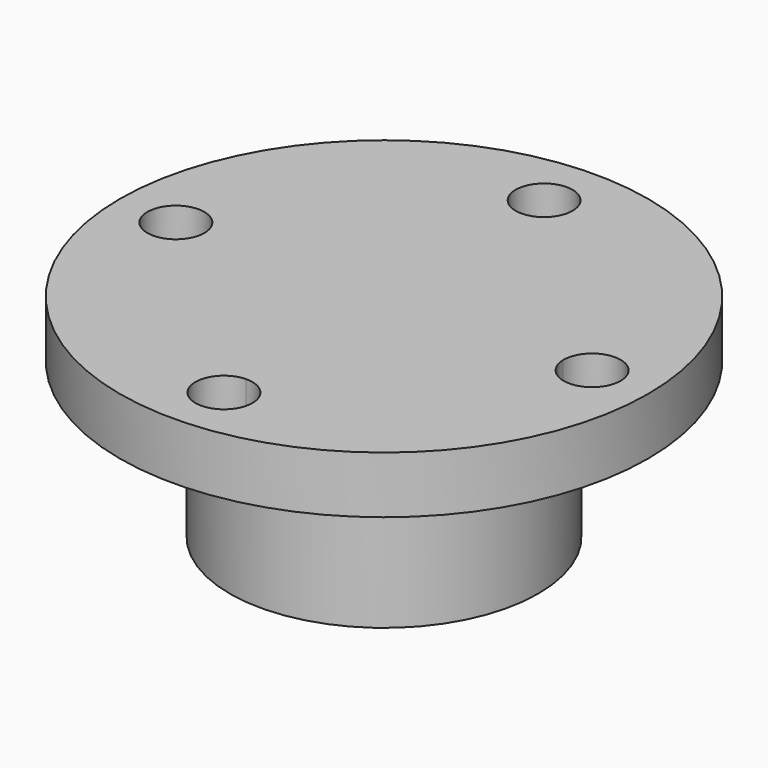
from build123d import *

# Parameters (mm, degrees)
F0_R         = 12.0396
F0_R_2       = 10.7696
F1_DEPTH     = 12.065
F2_R         = 20.6121
F3_DEPTH     = 4.445
F5_DEPTH     = 16.511
F6_S5_R      = 12.0396
F6_T6_DEPTH  = 7
F6_S11_R     = 12.0396
F6_T12_DEPTH = 7
F6_S17_R     = 12.0396
F6_T18_DEPTH = 7
F6_S23_R     = 12.0396
F6_T24_DEPTH = 7
F7_W         = 10.7836972851
F7_H         = 1.905
F7_W_2       = 1.905
F7_H_2       = 10.8237928489
F7_W_3       = 10.1713027149
F7_H_3       = 10.1312071511
F8_DEPTH     = 2.54


# Not quite as in the source:
# - a fillet or chamfer that OpenCascade refuses, or shapes differently, is made with other operations: its cross-section is extruded or revolved along the edge and cut away or added


with BuildPart() as f1:
    # F0 (on Top) → F1 (new body)
    with BuildSketch(Plane.XY):
        with Locations((-31.5266512334, -46.8901731074)):
            Circle(F0_R)
        with Locations((-31.5266512334, -46.8901731074)):
            Circle(F0_R_2, mode=Mode.SUBTRACT)
    extrude(amount=F1_DEPTH)

    # F2 (on face) → F3 (join)
    with BuildSketch(Plane.XY.offset(12.065)):
        with Locations((-31.5266512334, -46.8901731074)):
            Circle(F2_R)
    extrude(amount=F3_DEPTH)

    # F4 (on face) → F5 (cut, through all)
    with BuildSketch(Plane.XY.offset(16.51)):
        with BuildLine():
            ThreePointArc((-31.7884928641, -33.1131611233), (-30.2443193797, -32.4476041714), (-29.6082253852, -30.8910624162))
            ThreePointArc((-29.6082253852, -30.8910624162), (-33.4171313906, -29.3345206609), (-31.7884928641, -33.1131611233))
        make_face()
        with BuildLine():
            ThreePointArc((-13.3019866134, -46.5860989557), (-15.5486867731, -44.3606454902), (-17.7526926267, -46.6283895083))
            ThreePointArc((-17.7526926267, -46.6283895083), (-15.5063943113, -48.8115524211), (-13.3019866134, -46.5860989557))
        make_face()
        with BuildLine():
            ThreePointArc((-28.9935999678, -62.8892183723), (-29.6606432601, -61.3004657527), (-31.2619205449, -60.6640753873))
            ThreePointArc((-31.2619205449, -60.6640753873), (-32.777664533, -64.4779709918), (-28.9935999678, -62.8892183723))
        make_face()
        with BuildLine():
            ThreePointArc((-45.3002079959, -47.1942472591), (-45.3003084592, -47.1731010282), (-45.3006098402, -47.1519567065))
            ThreePointArc((-45.3006098402, -47.1519567065), (-49.7512153901, -47.21539349), (-45.3002079959, -47.1942472591))
        make_face()
    extrude(amount=-F5_DEPTH, mode=Mode.SUBTRACT)

    # F6: chamfer of 1.905 on 4 edges, made by hand


with BuildPart() as f6_tool2:
    # F6_s3 → F6_t4 (revolve)
    with BuildSketch(Plane.XZ.offset(62.8892183723)):
        Polygon((-27.0885999678, 12.065), (-28.9935999678, 13.97), (-28.9935999678, 12.065), align=None)
    revolve(axis=Axis((-31.2191538966, -62.8892183723, 12.065), (0, 0, 1)))

    # F6_s5 → F6_t6 (cut, symmetric)
    with BuildSketch(Plane.XY.offset(13)):
        with Locations((-31.5266512334, -46.8901731074)):
            Circle(F6_S5_R)
    extrude(amount=F6_T6_DEPTH, both=True, mode=Mode.SUBTRACT)


with BuildPart() as f1_1:
    add(f1.part)

    # F6_t1: cut F6_tool2
    add(f6_tool2.part, mode=Mode.SUBTRACT)


with BuildPart() as f6_tool8:
    # F6_s9 → F6_t10 (revolve)
    with BuildSketch(Plane.XZ.offset(46.5860989557)):
        Polygon((-11.3969866134, 12.065), (-13.3019866134, 13.97), (-13.3019866134, 12.065), align=None)
    revolve(axis=Axis((-15.5275405422, -46.5860989557, 12.065), (0, 0, 1)))

    # F6_s11 → F6_t12 (cut, symmetric)
    with BuildSketch(Plane.XY.offset(13)):
        with Locations((-31.5266512334, -46.8901731074)):
            Circle(F6_S11_R)
    extrude(amount=F6_T12_DEPTH, both=True, mode=Mode.SUBTRACT)


with BuildPart() as f1_2:
    add(f1_1.part)

    # F6_t7: cut F6_tool8
    add(f6_tool8.part, mode=Mode.SUBTRACT)


with BuildPart() as f6_tool14:
    # F6_s15 → F6_t16 (revolve)
    with BuildSketch(Plane(origin=(0.8794745138, -46.2742722997, 0), x_dir=(0, 0, 1), z_dir=(0.0190022592, -0.9998194408, 0))):
        Polygon((12.065, 44.2834241002), (13.97, 46.1884241002), (12.065, 46.1884241002), align=None)
    revolve(axis=Axis((-47.5257619247, -47.1942472591, 12.065), (0, 0, 1)))

    # F6_s17 → F6_t18 (cut, symmetric)
    with BuildSketch(Plane.XY.offset(13)):
        with Locations((-31.5266512334, -46.8901731074)):
            Circle(F6_S17_R)
    extrude(amount=F6_T18_DEPTH, both=True, mode=Mode.SUBTRACT)


with BuildPart() as f1_3:
    add(f1_2.part)

    # F6_t13: cut F6_tool14
    add(f6_tool14.part, mode=Mode.SUBTRACT)


with BuildPart() as f6_tool20:
    # F6_s21 → F6_t22 (revolve)
    with BuildSketch(Plane(origin=(-32.4061257472, -0.6159008077, 0), x_dir=(0, 0, 1), z_dir=(-0.9998194408, -0.0190022592, 0))):
        Polygon((12.065, -34.4081290555), (13.97, -32.5031290555), (12.065, -32.5031290555), align=None)
    revolve(axis=Axis((-31.8307253852, -30.8910624162, 12.065), (0, 0, 1)))

    # F6_s23 → F6_t24 (cut, symmetric)
    with BuildSketch(Plane.XY.offset(13)):
        with Locations((-31.5266512334, -46.8901731074)):
            Circle(F6_S23_R)
    extrude(amount=F6_T24_DEPTH, both=True, mode=Mode.SUBTRACT)


with BuildPart() as f1_4:
    add(f1_3.part)

    # F6_t19: cut F6_tool20
    add(f6_tool20.part, mode=Mode.SUBTRACT)

    # F7 (on face) → F8 (join)
    with BuildSketch(Plane(origin=(0, 0, 12.065), x_dir=(1, 0, 0), z_dir=(0, 0, -1))):
        with Locations((-37.7473032813, 46.6444636265)):
            Rectangle(F7_W, F7_H)
        with Locations((-31.4029546387, 53.008860051)):
            Rectangle(F7_W_2, F7_H_2)
        with Locations((-31.4029546387, 46.6444636265)):
            Rectangle(F7_W_2, F7_H)
        with Locations((-25.3648032813, 46.6444636265)):
            Rectangle(F7_W_3, F7_H)
        with Locations((-31.4029546387, 40.626360051)):
            Rectangle(F7_W_2, F7_H_3)
    extrude(amount=F8_DEPTH)


solid = f1_4.part
